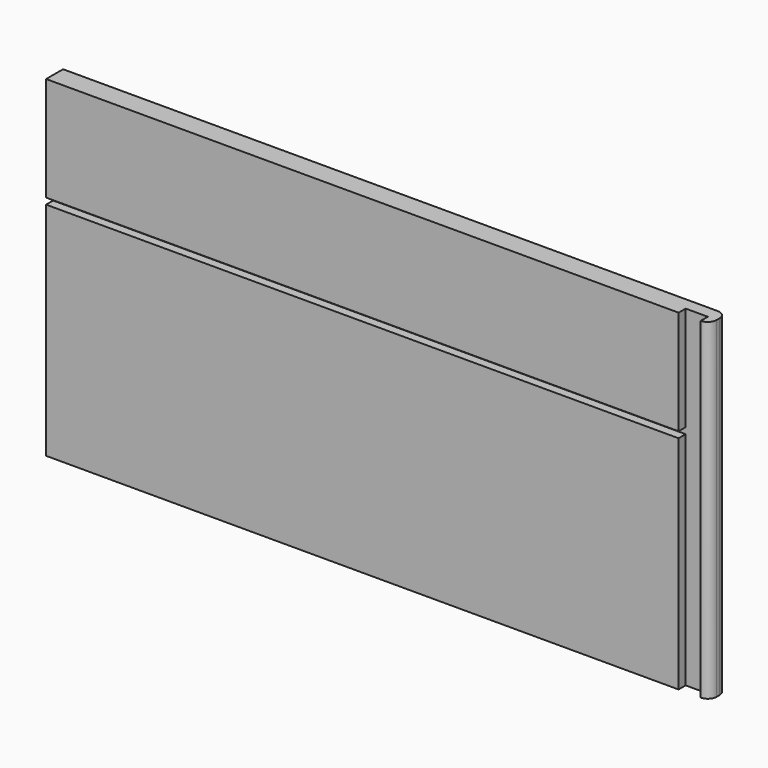
from build123d import *

# Parameters (mm, degrees)
F0_W     = 150
F0_H     = 75
F1_DEPTH = 4.8
F2_W     = 143
F2_H     = 1.4
F3_DEPTH = 2
F4_R     = 1.99999


# Not quite as in the source:
# - a fillet or chamfer is up to 0.001 mm smaller than in the source, because OpenCascade refuses the exact size


with BuildPart() as f1:
    # F0 (on Front) → F1 (new body)
    with BuildSketch(Plane.XZ):
        Rectangle(F0_W, F0_H)
    extrude(amount=F1_DEPTH)

    # F2 (on face) → F3 (cut)
    with BuildSketch(Plane.XZ.offset(4.8)):
        Polygon((68, 12.5), (68, -37.5), (73, -37.5), (73, 37.5), (68, 37.5), (68, 13.9), align=None)
        with Locations((-3.5, 13.2)):
            Rectangle(F2_W, F2_H)
    extrude(amount=-F3_DEPTH, mode=Mode.SUBTRACT)

    # F4 (radius 2 in the source; OpenCascade refuses exactly that, so slightly less here)
    f4_edges = [f1.edges().sort_by_distance(p)[0] for p in [
        (75, 0, 0),
        (75, -4.8, 0),
    ]]
    fillet(f4_edges, radius=F4_R)


solid = f1.part
